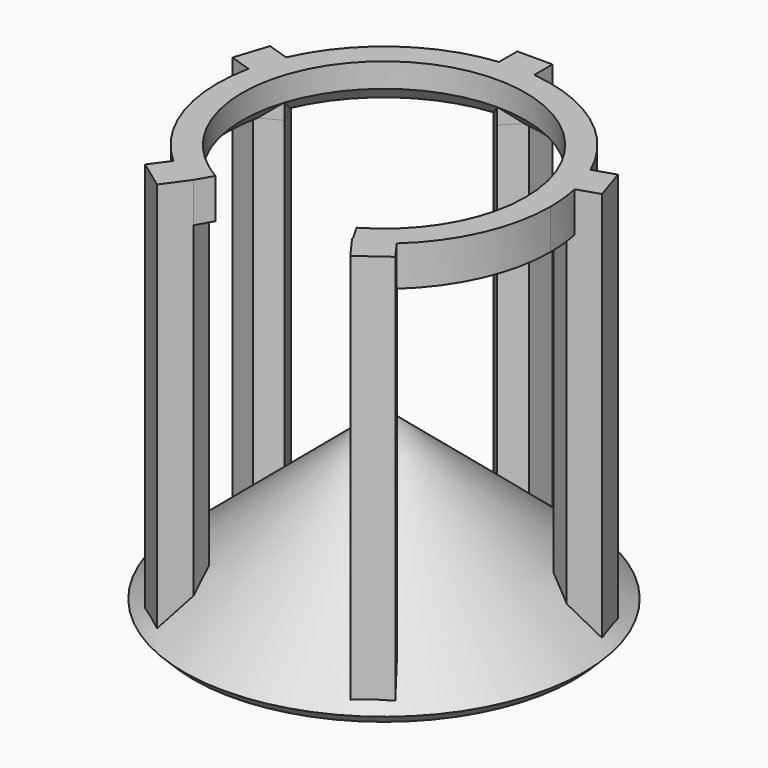
from build123d import *

# Parameters (mm, degrees)
F3_DEPTH     = 25.4
F5_DEPTH     = 2.54
F1_FACE_R    = 12.7
F6_DEPTH     = 0.6
F6_TAPER     = 45
F7_T4_ANGLE  = 71.9999997561
F7_T10_ANGLE = 72.000000061
F7_T16_ANGLE = 72.000000061
F7_T22_ANGLE = 72.000000061


# Not quite as in the source:
# - a fillet or chamfer that OpenCascade refuses, or shapes differently, is made with other operations: its cross-section is extruded or revolved along the edge and cut away or added


with BuildPart() as f1:
    # F0 (on Front) → F1 (revolve)
    with BuildSketch(Plane.XZ):
        Polygon((0, 10.656565316), (0, 0), (12.7, 0), align=None)
    revolve(axis=Axis((0, 0, 24.9413493462), (0, 0, 1)))

    # F2 (on Top) → F3 (join)
    with BuildSketch(Plane.XY):
        Polygon((-9.9684698397, 2.0625815326), (-8.5595086348, 2.7811529858), (-9.2770164791, 4.1906561266), (-11.0598678693, 4.7699396671), (-11.7513212299, 2.6418650731), align=None)
        Polygon((-1.1187950245, 10.1179509397), (0, 9), (1.1187950245, 10.1179509397), (1.1187950245, 11.9925518305), (-1.1187950245, 11.9925518305), align=None)
        Polygon((9.2770165014, 4.1906560772), (8.5595086496, 2.7811529403), (9.9684698507, 2.0625814795), (11.751321244, 2.6418650106), (11.0598678947, 4.7699396082), align=None)
        Polygon((6.8523065178, -7.5279830573), (5.2900672551, -7.2811529606), (5.0420581389, -8.8432054849), (6.1439208932, -10.3597894656), (7.9541692721, -9.044567038), align=None)
        Polygon((-5.0420581859, -8.8432054581), (-5.2900672939, -7.2811529325), (-6.8523065578, -7.5279830208), (-7.9541693202, -9.0445669956), (-6.1439209483, -10.3597894329), align=None)
    extrude(amount=F3_DEPTH)

    # F4 (on face) → F5 (join)
    with BuildSketch(Plane.XY.offset(25.4)):
        with BuildLine():
            ThreePointArc((-5.2900672939, -7.2811529325), (-4.0859144849, 8.0190587242), (9, 0))
            ThreePointArc((9, 0), (7.7919238303, -4.5039896783), (4.4920171062, -7.7988321124))
            Line((4.4920171062, -7.7988321124), (5.2905979251, -9.1852911546))
            ThreePointArc((5.2905979251, -9.1852911546), (9.1771547335, -5.3046989544), (10.6, 0))
            ThreePointArc((10.6, 0), (-4.306450321, 9.6857878168), (-7.1008463458, -7.8700686892))
            Line((-7.1008463458, -7.8700686892), (-6.8523065578, -7.5279830208))
            Line((-6.8523065578, -7.5279830208), (-5.2900672939, -7.2811529325))
        make_face()
        with BuildLine():
            ThreePointArc((-4.457782334, -7.8184510399), (-4.8813231204, -7.5612621033), (-5.2900672939, -7.2811529325))
            Line((-5.2900672939, -7.2811529325), (-5.0420581859, -8.8432054581))
            Line((-5.0420581859, -8.8432054581), (-4.457782334, -7.8184510399))
        make_face()
    extrude(amount=-F5_DEPTH)

    # F1_face (on face) → F6 (join)
    with BuildSketch(Plane(origin=(0, 0, 0), x_dir=(1, 0, 0), z_dir=(0, 0, -1))):
        Circle(F1_FACE_R)
    extrude(amount=F6_DEPTH, taper=F6_TAPER)

    # F7: chamfer of 1 on 4 edges, made by hand


with BuildPart() as f7_tool2:
    # F7_s3 → F7_t4 (revolve)
    with BuildSketch(Plane(origin=(0, 0, 0), x_dir=(0, 0, 1), z_dir=(-0.3090169984, -0.951056515, 0))):
        Polygon((22.86, 10), (23.86, 9), (22.86, 9), align=None)
    revolve(axis=Axis((0, 0, 22.86), (0, 0, -1)), revolution_arc=F7_T4_ANGLE)

    split(bisect_by=Plane(origin=(4.4999987183, 4.5033963456, 0), x_dir=(0, 0, 1), z_dir=(-0.7068398887, -0.707373573, 0)), keep=Keep.TOP)

    split(bisect_by=Plane(origin=(-5.6735605309, -2.888127077, 0), x_dir=(0, 0, 1), z_dir=(0.8911777859, 0.4536542229, 0)), keep=Keep.TOP)


with BuildPart() as f1_1:
    add(f1.part)

    # F7_t1: cut F7_tool2
    add(f7_tool2.part, mode=Mode.SUBTRACT)


with BuildPart() as f7_tool8:
    # F7_s9 → F7_t10 (revolve)
    with BuildSketch(Plane(origin=(0, 0, 0), x_dir=(0, 0, 1), z_dir=(0.8090169925, -0.5877852549, 0))):
        Polygon((22.86, 10), (23.86, 9), (22.86, 9), align=None)
    revolve(axis=Axis((0, 0, 22.86), (0, 0, -1)), revolution_arc=F7_T10_ANGLE)

    split(bisect_by=Plane(origin=(-2.8924083372, 5.6713791199, 0), x_dir=(0, 0, 1), z_dir=(0.4543267043, -0.8908351395, 0)), keep=Keep.TOP)

    split(bisect_by=Plane(origin=(0.9935454605, -6.2883570612, 0), x_dir=(0, 0, 1), z_dir=(-0.1560617251, 0.9877473047, 0)), keep=Keep.TOP)


with BuildPart() as f1_2:
    add(f1_1.part)

    # F7_t7: cut F7_tool8
    add(f7_tool8.part, mode=Mode.SUBTRACT)


with BuildPart() as f7_tool14:
    # F7_s15 → F7_t16 (revolve)
    with BuildSketch(Plane.YZ):
        Polygon((10, 22.86), (9, 23.86), (9, 22.86), align=None)
    revolve(axis=Axis((0, 0, 22.86), (0, 0, -1)), revolution_arc=F7_T16_ANGLE)

    split(bisect_by=Plane(origin=(5.6735605155, -2.8881271072, 0), x_dir=(0, 0, 1), z_dir=(-0.8911777835, 0.4536542277, 0)), keep=Keep.TOP)

    split(bisect_by=Plane(origin=(-4.4999987183, 4.5033963456, 0), x_dir=(0, 0, 1), z_dir=(0.7068398887, -0.707373573, 0)), keep=Keep.TOP)


with BuildPart() as f1_3:
    add(f1_2.part)

    # F7_t13: cut F7_tool14
    add(f7_tool14.part, mode=Mode.SUBTRACT)


with BuildPart() as f7_tool20:
    # F7_s21 → F7_t22 (revolve)
    with BuildSketch(Plane(origin=(0, 0, 0), x_dir=(0, 0, 1), z_dir=(-0.3090169934, 0.9510565166, 0))):
        Polygon((22.86, 10), (23.86, 9), (22.86, 9), align=None)
    revolve(axis=Axis((0, 0, 22.86), (0, 0, -1)), revolution_arc=F7_T22_ANGLE)

    split(bisect_by=Plane(origin=(2.8924083674, 5.6713791045, 0), x_dir=(0, 0, 1), z_dir=(-0.4543267091, -0.8908351371, 0)), keep=Keep.TOP)

    split(bisect_by=Plane(origin=(-0.993545494, -6.2883570559, 0), x_dir=(0, 0, 1), z_dir=(0.1560617303, 0.9877473039, 0)), keep=Keep.TOP)


with BuildPart() as f1_4:
    add(f1_3.part)

    # F7_t19: cut F7_tool20
    add(f7_tool20.part, mode=Mode.SUBTRACT)


solid = f1_4.part
